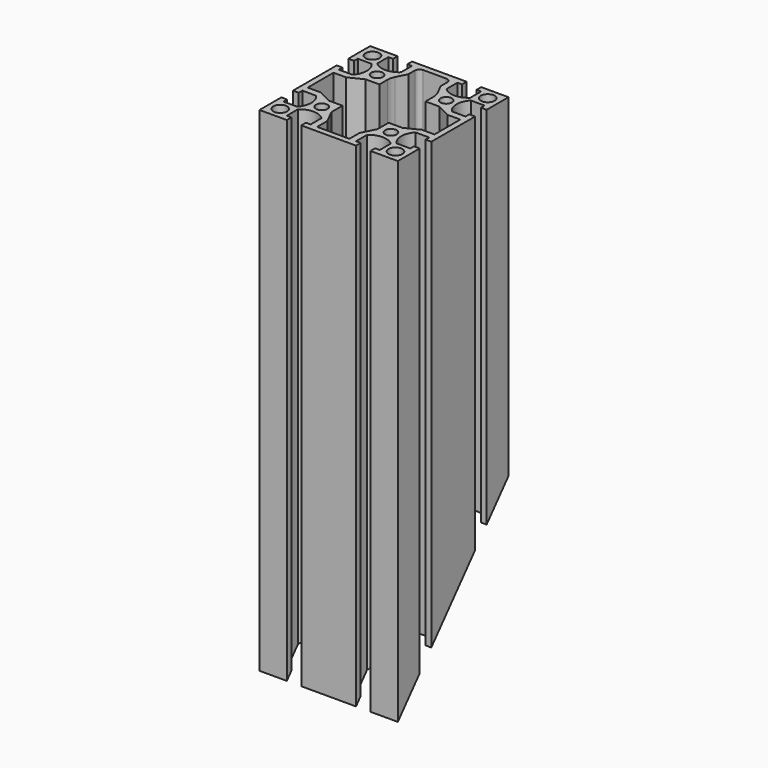
from build123d import *

# Parameters (mm, degrees)
F0_R          = 3
F0_R_2        = 2.5
F1_DEPTH      = 214.17
F2_R          = 2
F3_R          = 7
F5_DEPTH      = 30
F5_DEPTH_BACK = 30


# Not quite as in the source:
# - a feature names something its author has since deleted; it is built from what else it names


with BuildPart() as f1:
    # F0 (on Top) → F1 (new body)
    with BuildSketch(Plane.XY):
        with BuildLine():
            Line((18.15, -30), (30, -30))
            Line((30, -30), (30, -18.15))
            Line((30, -18.15), (27.5, -18.15))
            Line((27.5, -18.15), (27.5, -20.15))
            Line((27.5, -20.15), (21.5477069044, -20.15))
            ThreePointArc((21.5477069044, -20.15), (19.5, -15), (21.5477069044, -9.85))
            Line((21.5477069044, -9.85), (27.5, -9.85))
            Line((27.5, -9.85), (27.5, -11.85))
            Line((27.5, -11.85), (30, -11.85))
            Line((30, -11.85), (30, 11.85))
            Line((30, 11.85), (27.5, 11.85))
            Line((27.5, 11.85), (27.5, 9.85))
            Line((27.5, 9.85), (21.5477069044, 9.85))
            ThreePointArc((21.5477069044, 9.85), (19.5, 15), (21.5477069044, 20.15))
            Line((21.5477069044, 20.15), (27.5, 20.15))
            Line((27.5, 20.15), (27.5, 18.15))
            Line((27.5, 18.15), (30, 18.15))
            Line((30, 18.15), (30, 30))
            Line((30, 30), (18.15, 30))
            Line((18.15, 30), (18.15, 27.5))
            Line((18.15, 27.5), (20.15, 27.5))
            Line((20.15, 27.5), (20.15, 21.5477069044))
            ThreePointArc((20.15, 21.5477069044), (15, 19.5), (9.85, 21.5477069044))
            Line((9.85, 21.5477069044), (9.85, 27.5))
            Line((9.85, 27.5), (11.85, 27.5))
            Line((11.85, 27.5), (11.85, 30))
            Line((11.85, 30), (-11.85, 30))
            Line((-11.85, 30), (-11.85, 27.5))
            Line((-11.85, 27.5), (-9.85, 27.5))
            Line((-9.85, 27.5), (-9.85, 21.5477069044))
            ThreePointArc((-9.85, 21.5477069044), (-15, 19.5), (-20.15, 21.5477069044))
            Line((-20.15, 21.5477069044), (-20.15, 27.5))
            Line((-20.15, 27.5), (-18.15, 27.5))
            Line((-18.15, 27.5), (-18.15, 30))
            Line((-18.15, 30), (-30, 30))
            Line((-30, 30), (-30, 18.15))
            Line((-30, 18.15), (-27.5, 18.15))
            Line((-27.5, 18.15), (-27.5, 20.15))
            Line((-27.5, 20.15), (-21.5477069044, 20.15))
            ThreePointArc((-21.5477069044, 20.15), (-19.5, 15), (-21.5477069044, 9.85))
            Line((-21.5477069044, 9.85), (-27.5, 9.85))
            Line((-27.5, 9.85), (-27.5, 11.85))
            Line((-27.5, 11.85), (-30, 11.85))
            Line((-30, 11.85), (-30, -11.85))
            Line((-30, -11.85), (-27.5, -11.85))
            Line((-27.5, -11.85), (-27.5, -9.85))
            Line((-27.5, -9.85), (-21.5477069044, -9.85))
            ThreePointArc((-21.5477069044, -9.85), (-19.5, -15), (-21.5477069044, -20.15))
            Line((-21.5477069044, -20.15), (-27.5, -20.15))
            Line((-27.5, -20.15), (-27.5, -18.15))
            Line((-27.5, -18.15), (-30, -18.15))
            Line((-30, -18.15), (-30, -30))
            Line((-30, -30), (-18.15, -30))
            Line((-18.15, -30), (-18.15, -27.5))
            Line((-18.15, -27.5), (-20.15, -27.5))
            Line((-20.15, -27.5), (-20.15, -21.5477069044))
            ThreePointArc((-20.15, -21.5477069044), (-15, -19.5), (-9.85, -21.5477069044))
            Line((-9.85, -21.5477069044), (-9.85, -27.5))
            Line((-9.85, -27.5), (-11.85, -27.5))
            Line((-11.85, -27.5), (-11.85, -30))
            Line((-11.85, -30), (11.85, -30))
            Line((11.85, -30), (11.85, -27.5))
            Line((11.85, -27.5), (9.85, -27.5))
            Line((9.85, -27.5), (9.85, -21.5477069044))
            ThreePointArc((9.85, -21.5477069044), (15, -19.5), (20.15, -21.5477069044))
            Line((20.15, -21.5477069044), (20.15, -27.5))
            Line((20.15, -27.5), (18.15, -27.5))
            Line((18.15, -27.5), (18.15, -30))
        make_face()
        with Locations((-25, -25)):
            Circle(F0_R, mode=Mode.SUBTRACT)
        with Locations((-15, -15)):
            Circle(F0_R_2, mode=Mode.SUBTRACT)
        with Locations((25, -25)):
            Circle(F0_R, mode=Mode.SUBTRACT)
        with Locations((15, -15)):
            Circle(F0_R_2, mode=Mode.SUBTRACT)
        with Locations((-25, 25)):
            Circle(F0_R, mode=Mode.SUBTRACT)
        with Locations((-15, 15)):
            Circle(F0_R_2, mode=Mode.SUBTRACT)
        Polygon((-7, 22), (-7, 27.5), (0, 27.5), (7, 27.5), (7, 22), (10, 16), (10, 10), (16, 10), (22, 7), (27.5, 7), (27.5, 0), (27.5, -7), (22, -7), (16, -10), (10, -10), (10, -16), (7, -22), (7, -27.5), (0, -27.5), (-7, -27.5), (-7, -22), (-10, -16), (-10, -10), (-16, -10), (-22, -7), (-27.5, -7), (-27.5, 0), (-27.5, 7), (-22, 7), (-16, 10), (-10, 10), (-10, 16), align=None, mode=Mode.SUBTRACT)
        with Locations((15, 15)):
            Circle(F0_R_2, mode=Mode.SUBTRACT)
        with Locations((25, 25)):
            Circle(F0_R, mode=Mode.SUBTRACT)
    extrude(amount=F1_DEPTH)

    # F2
    f2_edges = [f1.edges().sort_by_distance(p)[0] for p in [
        (-7, 27.5, 107.085),
        (7, 27.5, 107.085),
    ]]
    fillet(f2_edges, radius=F2_R)

    # F3
    f3_edges = [f1.edges().sort_by_distance(p)[0] for p in [
        (-10, 16, 107.085),
        (10, 16, 107.085),
    ]]
    fillet(f3_edges, radius=F3_R)

    # F4 (on Right) → F5 (cut, two sides)
    with BuildSketch(Plane.YZ) as f5_sk:
        Polygon((71.6507620084, 117.7635412378), (-30, 0), (52.6850404625, -71.3718123739), (154.335802471, 46.3917288639), align=None)
    extrude(amount=F5_DEPTH, mode=Mode.SUBTRACT)
    extrude(f5_sk.sketch, amount=-F5_DEPTH_BACK, mode=Mode.SUBTRACT)


solid = f1.part
